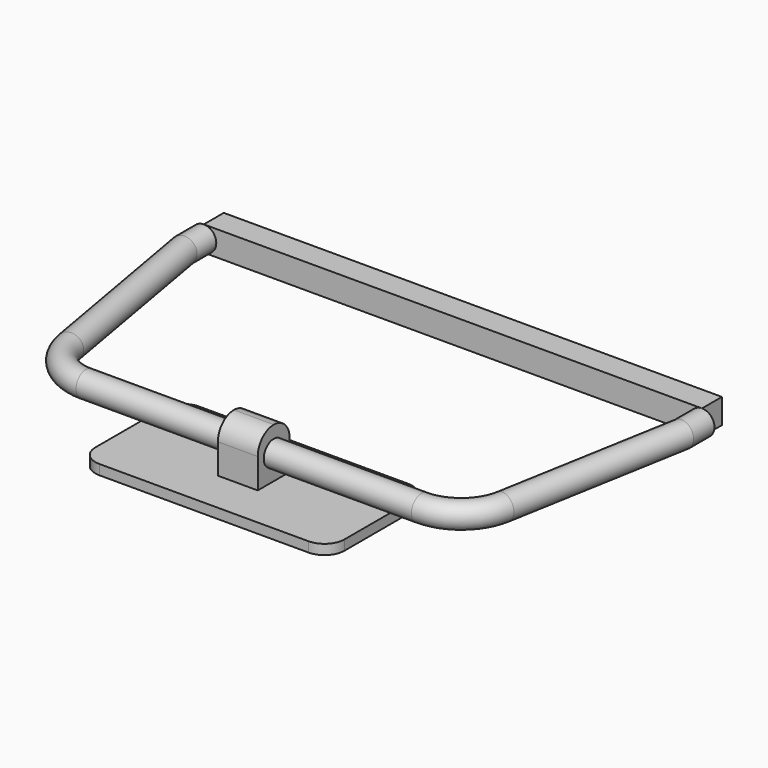
from build123d import *

# Parameters (mm, degrees)
F0_R          = 12.5
F4_DEPTH      = 25
F5_W          = 40
F5_H          = 40
F6_DEPTH      = 25
F6_DEPTH_BACK = 25
F7_R          = 19.99999
F9_DEPTH      = 10


# Not quite as in the source:
# - a fillet or chamfer is up to 0.001 mm smaller than in the source, because OpenCascade refuses the exact size


with BuildPart() as f2:
    # F2: sweep along a path in F1
    with BuildLine(Plane.XY) as f2_path:
        Line((-465.6524967789, 0), (-465.6524967789, -25))
        Line((-465.6524967789, -25), (-433.2643322113, -208.6824088833))
        ThreePointArc((-433.2643322113, -208.6824088833), (-416.163325045, -238.3022221559), (-384.0239445606, -250))
        Line((-384.0239445606, -250), (-47.2810489972, -250))
        ThreePointArc((-47.2810489972, -250), (-15.1416685129, -238.3022221559), (1.9593386534, -208.6824088833))
        Line((1.9593386534, -208.6824088833), (34.3475032211, -25))
        Line((34.3475032211, -25), (34.3475032211, 0))
    # F0 (on Front) → F2 (sweep)
    with BuildSketch(Plane.XZ):
        with Locations((-465.6524967789, 0)):
            Circle(F0_R)
    sweep(path=f2_path.line, transition=Transition.RIGHT)

    # F3 (on face) → F4 (join)
    with BuildSketch(Plane(origin=(0, 0, 0), x_dir=(-1, 0, 0), z_dir=(0, 1, 0))):
        with BuildLine():
            Line((465.6524967789, 12.5), (-34.3475032211, 12.5))
            Line((-34.3475032211, 12.5), (-34.3475032211, -12.5))
            Line((-34.3475032211, -12.5), (465.6524967789, -12.5))
            ThreePointArc((465.6524967789, -12.5), (453.1524967789, 0), (465.6524967789, 12.5))
        make_face()
        with BuildLine():
            Line((465.6524967789, -12.5), (465.6524967789, 12.5))
            ThreePointArc((465.6524967789, 12.5), (453.1524967789, 0), (465.6524967789, -12.5))
        make_face()
    extrude(amount=F4_DEPTH)

    # F5 (on Top) → F6 (join, two sides)
    with BuildSketch(Plane.XY) as f6_sk:
        with Locations((-215.5239445606, -250)):
            Rectangle(F5_W, F5_H)
    extrude(amount=F6_DEPTH)
    extrude(f6_sk.sketch, amount=-F6_DEPTH_BACK)

    # F7 (radius 20 in the source; OpenCascade refuses exactly that, so slightly less here)
    f7_edges = [f2.edges().sort_by_distance(p)[0] for p in [
        (-215.523945, -230, 25),
        (-215.523945, -270, 25),
    ]]
    fillet(f7_edges, radius=F7_R)

    # F8 (on face) → F9 (join)
    with BuildSketch(Plane(origin=(0, 0, -25), x_dir=(1, 0, 0), z_dir=(0, 0, -1))):
        with BuildLine():
            Line((-110.5239445606, 312.5), (-320.5239445606, 312.5))
            ThreePointArc((-320.5239445606, 312.5), (-334.6660801844, 306.6421356237), (-340.5239445606, 292.5))
            Line((-340.5239445606, 292.5), (-340.5239445606, 207.5))
            ThreePointArc((-340.5239445606, 207.5), (-334.6660801844, 193.3578643763), (-320.5239445606, 187.5))
            Line((-320.5239445606, 187.5), (-110.5239445606, 187.5))
            ThreePointArc((-110.5239445606, 187.5), (-96.3818089369, 193.3578643763), (-90.5239445606, 207.5))
            Line((-90.5239445606, 207.5), (-90.5239445606, 292.5))
            ThreePointArc((-90.5239445606, 292.5), (-96.3818089369, 306.6421356237), (-110.5239445606, 312.5))
        make_face()
    extrude(amount=F9_DEPTH)


solid = f2.part
